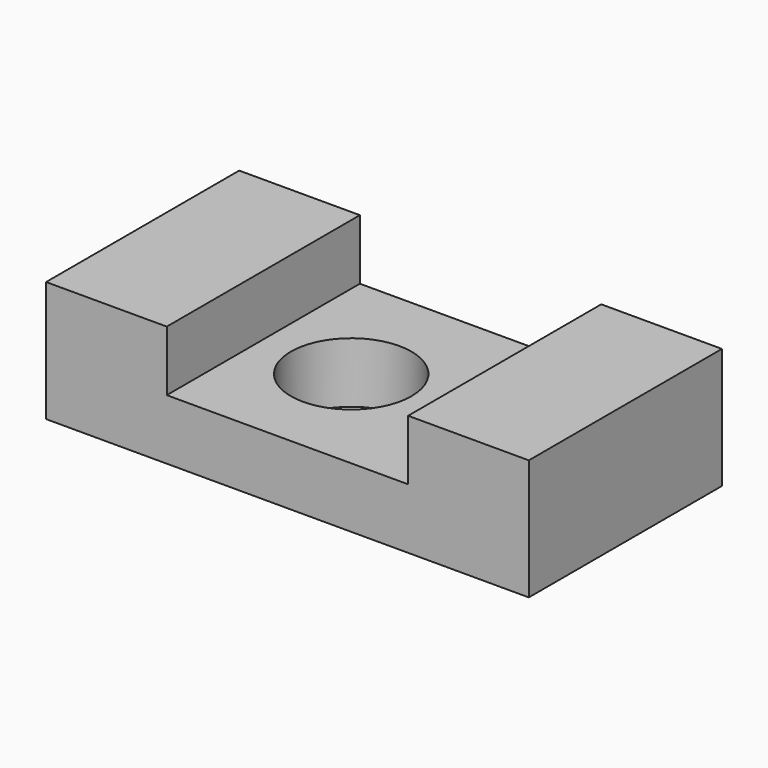
from build123d import *

# Parameters (mm, degrees)
F0_W     = 200
F0_H     = 100
F0_R     = 25
F1_DEPTH = 50
F2_W     = 100
F2_H     = 100
F2_R     = 25
F3_DEPTH = 25


# Not quite as in the source:
# - a feature names something its author has since deleted; it is built from what else it names


with BuildPart() as f1:
    # F0 (on Top) → F1 (new body)
    with BuildSketch(Plane.XY):
        with Locations((12.7213582092, 1.0950192809)):
            Rectangle(F0_W, F0_H)
        Circle(F0_R, mode=Mode.SUBTRACT)
    extrude(amount=F1_DEPTH)

    # F2 (on face) → F3 (cut)
    with BuildSketch(Plane.XY.offset(50)):
        with Locations((12.7213582092, 1.0950192809)):
            Rectangle(F2_W, F2_H)
        Circle(F2_R, mode=Mode.SUBTRACT)
    extrude(amount=-F3_DEPTH, mode=Mode.SUBTRACT)


solid = f1.part
